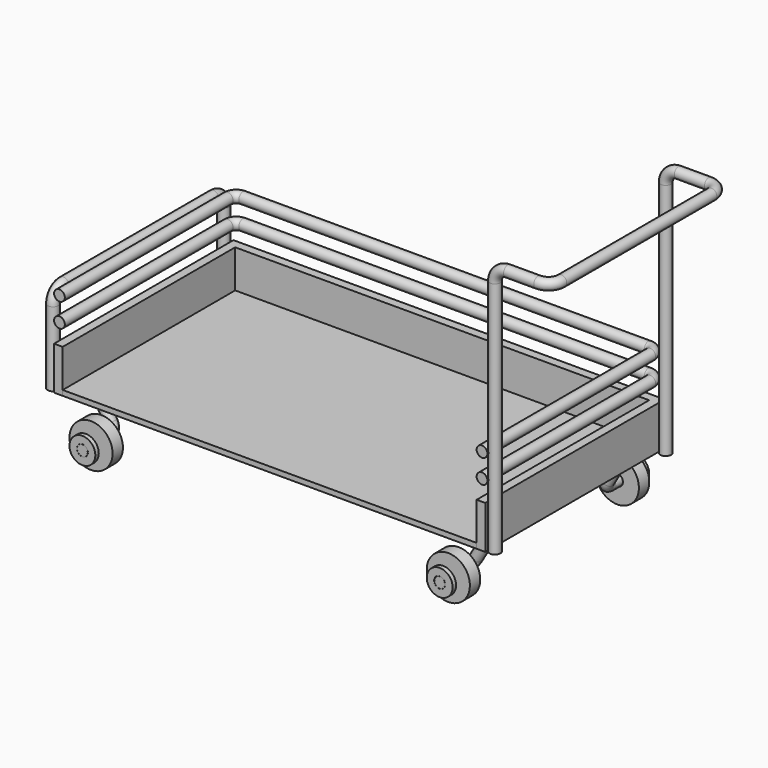
from build123d import *

# Parameters (mm, degrees)
F0_W      = 96
F0_H      = 50
F1_DEPTH  = 1.2
F3_DEPTH  = 10
F5_R      = 1.25
F9_R      = 1.25
F13_R     = 1.25
F4_R      = 1.25
F29_R     = 1.25
F32_R     = 3
F32_R_2   = 1.275
F33_DEPTH = 1
F34_R     = 5
F34_R_2   = 1.3
F35_DEPTH = 3


with BuildPart() as f1:
    # F0 (on Top) → F1 (new body)
    with BuildSketch(Plane.XY):
        Rectangle(F0_W, F0_H)
    extrude(amount=F1_DEPTH)

    # F30: sweep along a path in F27
    with BuildLine(Plane(origin=(-34.5428847577, 0, -19.9433438135), x_dir=(0, 1, 0), z_dir=(0.8660254038, 0, 0.5))) as f30_path:
        Line((-27.5, 13.7785898385), (-20, 13.7785898385))
        ThreePointArc((-20, 13.7785898385), (-18.5857864376, 14.3643762761), (-18, 15.7785898385))
        Line((-18, 15.7785898385), (-18, 19.7785898385))
        ThreePointArc((-18, 19.7785898385), (-17.4142135624, 21.1928034009), (-16, 21.7785898385))
        Line((-16, 21.7785898385), (18, 21.7785898385))
        ThreePointArc((18, 21.7785898385), (19.4142135624, 21.1928034009), (20, 19.7785898385))
        Line((20, 19.7785898385), (20, 15.7785898385))
        ThreePointArc((20, 15.7785898385), (20.5857864376, 14.3643762761), (22, 13.7785898385))
        Line((22, 13.7785898385), (29.5, 13.7785898385))
    # F29 (on line) → F30 (sweep)
    with BuildSketch(Plane.XZ.offset(27.5)):
        with Locations((-41.432179677, -8.010734985)):
            Circle(F29_R)
    sweep(path=f30_path.line)

    # F31: F1 across plane


with BuildPart() as f3:
    # F2 (on Top) → F3 (new body)
    with BuildSketch(Plane.XY):
        Polygon((-48, -25), (-48, 25), (48, 25), (48, -25), (50, -25), (50, 27), (-50, 27), (-50, -25), align=None)
    extrude(amount=F3_DEPTH)


with BuildPart() as f8:
    # F8: sweep along a path in F7
    with BuildLine(Plane.YZ.offset(-51.25)) as f8_path:
        Line((-23.75, 0), (-23.75, 17.25))
        ThreePointArc((-23.75, 17.25), (-22.8713203436, 19.3713203436), (-20.75, 20.25))
        Line((-20.75, 20.25), (22.75, 20.25))
        ThreePointArc((22.75, 20.25), (24.8713203436, 19.3713203436), (25.75, 17.25))
        Line((25.75, 17.25), (25.75, 0))
    # F5 (on Top) → F8 (sweep)
    with BuildSketch(Plane.XY):
        with Locations((-51.25, -23.75)):
            Circle(F5_R)
    sweep(path=f8_path.line)


with BuildPart() as f12:
    # F12: sweep along a path in F11
    with BuildLine(Plane.XY.offset(20.25)) as f12_path:
        Line((-48.75, -25), (-48.75, 23.75))
        ThreePointArc((-48.75, 23.75), (-48.1642135624, 25.1642135624), (-46.75, 25.75))
        Line((-46.75, 25.75), (47.25, 25.75))
        ThreePointArc((47.25, 25.75), (48.6642135624, 25.1642135624), (49.25, 23.75))
        Line((49.25, 23.75), (49.25, -25))
    # F9 (on face) → F12 (sweep)
    with BuildSketch(Plane.XZ.offset(25)):
        with Locations((-48.75, 20.25)):
            Circle(F9_R)
    sweep(path=f12_path.line)


with BuildPart() as f16:
    # F16: sweep along a path in F15
    with BuildLine(Plane.XY.offset(14.75)) as f16_path:
        Line((-48.75, -25), (-48.75, 23.75))
        ThreePointArc((-48.75, 23.75), (-48.1642135624, 25.1642135624), (-46.75, 25.75))
        Line((-46.75, 25.75), (47.25, 25.75))
        ThreePointArc((47.25, 25.75), (48.6642135624, 25.1642135624), (49.25, 23.75))
        Line((49.25, 23.75), (49.25, -25))
    # F13 (on face) → F16 (sweep)
    with BuildSketch(Plane.XZ.offset(25)):
        with Locations((-48.75, 14.75)):
            Circle(F13_R)
    sweep(path=f16_path.line)


with BuildPart() as f23:
    # F23: sweep along a path in F18, F22, F20
    with BuildLine(Plane.XZ.offset(23.75)) as f23_path:
        Line((51.25, 0), (51.25, 55.25))
        ThreePointArc((51.25, 55.25), (52.1286796564, 57.3713203436), (54.25, 58.25))
    with BuildLine(Plane.XY.offset(58.25)) as f23_path_2:
        Line((54.25, -23.75), (61.25, -23.75))
        ThreePointArc((61.25, -23.75), (63.3713203436, -22.8713203436), (64.25, -20.75))
        Line((64.25, -20.75), (64.25, 22.75))
        ThreePointArc((64.25, 22.75), (63.3713203436, 24.8713203436), (61.25, 25.75))
        Line((61.25, 25.75), (54.25, 25.75))
    with BuildLine(Plane(origin=(0, 25.75, 0), x_dir=(-1, 0, 0), z_dir=(0, 1, 0))) as f23_path_3:
        ThreePointArc((-54.25, 58.25), (-52.1286796564, 57.3713203436), (-51.25, 55.25))
        Line((-51.25, 55.25), (-51.25, 0))
    # F4 (on Top) → F23 (sweep)
    with BuildSketch(Plane.XY):
        with Locations((51.25, -23.75)):
            Circle(F4_R)
    sweep(path=f23_path.line + f23_path_2.line + f23_path_3.line)


with BuildPart() as f1_1:
    add(f1.part)
    add(f1.part.mirror(Plane.YZ))


with BuildPart() as f33:
    # F32 (on face) → F33 (new body)
    with BuildSketch(Plane.XZ.offset(27.5)):
        with Locations((-41.432179677, -8.010734985)):
            Circle(F32_R)
        with Locations((-41.432179677, -8.010734985)):
            Circle(F32_R_2, mode=Mode.SUBTRACT)
    extrude(amount=-F33_DEPTH)


with BuildPart() as f35:
    # F34 (on face) → F35 (new body)
    with BuildSketch(Plane.XZ.offset(25)):
        with Locations((-41.432179677, -8.010734985)):
            Circle(F34_R)
        with Locations((-41.432179677, -8.010734985)):
            Circle(F34_R_2, mode=Mode.SUBTRACT)
    extrude(amount=-F35_DEPTH)


with BuildPart() as f37_1:
    # F37: instance of F35
    add(f35.part.mirror(Plane.XZ.offset(-1)))


with BuildPart() as f37_2:
    # F37: instance of F33
    add(f33.part.mirror(Plane.XZ.offset(-1)))


with BuildPart() as f38_1:
    # F38: instance of F33
    add(f33.part.mirror(Plane.YZ))


with BuildPart() as f38_2:
    # F38: instance of F35
    add(f35.part.mirror(Plane.YZ))


with BuildPart() as f38_3:
    # F38: instance of F37_2
    add(f37_2.part.mirror(Plane.YZ))


with BuildPart() as f38_4:
    # F38: instance of F37_1
    add(f37_1.part.mirror(Plane.YZ))


solid = Compound([f3.part, f8.part, f12.part, f16.part, f23.part, f1_1.part, f33.part, f35.part, f37_1.part, f37_2.part, f38_1.part, f38_2.part, f38_3.part, f38_4.part])
